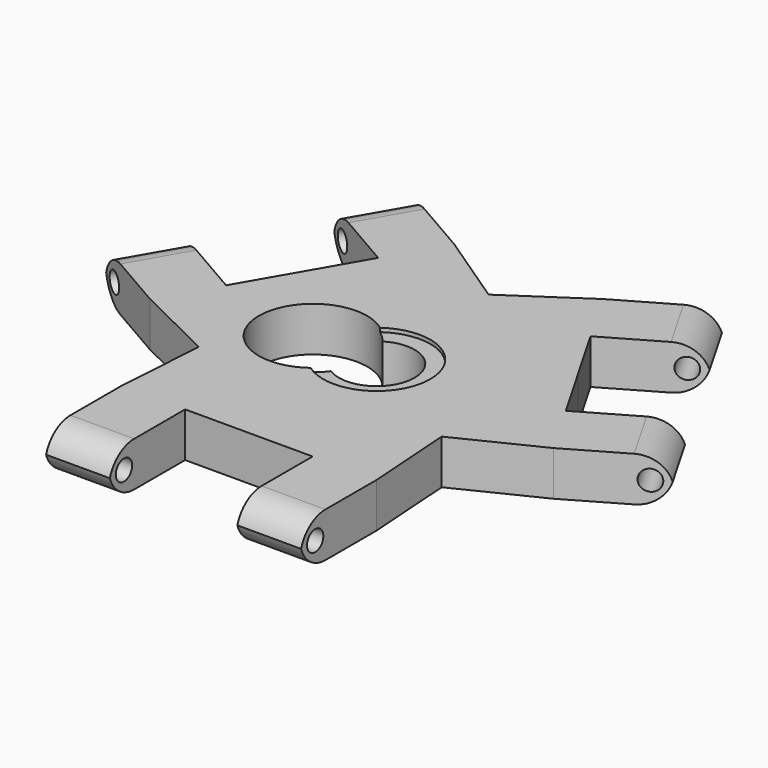
from build123d import *

# Parameters (mm, degrees)
F0_W         = 10
F0_H         = 15
F1_DEPTH     = 7
F3_DEPTH     = 60
F4_R         = 1.6
F5_DEPTH     = 60
F6_R         = 1.6
F7_DEPTH     = 60
F8_T1_DEPTH  = 35
F8_T3_DEPTH  = 35
F8_T5_DEPTH  = 35
F8_T7_DEPTH  = 35
F8_T9_DEPTH  = 35
F8_T11_DEPTH = 35
F11_DEPTH    = 25
F12_R        = 8.4
F13_DEPTH    = 0.6


# Not quite as in the source:
# - a fillet or chamfer that OpenCascade refuses, or shapes differently, is made with other operations: its cross-section is extruded or revolved along the edge and cut away or added
# - a feature names something its author has since deleted; it is built from what else it names


with BuildPart() as f1:
    # F0 (on Top) → F1 (new body)
    with BuildSketch(Plane.XY):
        Polygon((-19.0935776077, -11.020506829), (-0.0410187244, -0.020506829), (-21.6916538191, 12.479493171), (-26.6916538191, 3.8192391331), (-31.6916538191, -4.8410149047), align=None)
        Polygon((-0.0410187244, 21.979493171), (-0.0410187244, -0.020506829), (21.6096163702, 12.479493171), (16.6096163702, 21.1397472088), (11.6096163702, 29.8000012467), align=None)
        Polygon((19.0115401588, -11.020506829), (-0.0410187244, -0.020506829), (-0.0410187244, -25.020506829), (9.9589812756, -25.020506829), (19.9589812756, -25.020506829), align=None)
        Polygon((-0.0410187244, -25.020506829), (-0.0410187244, -0.020506829), (-19.0935776077, -11.020506829), (-20.0410187244, -25.020506829), (-10.0410187244, -25.020506829), align=None)
        Polygon((-21.6916538191, 12.479493171), (-0.0410187244, -0.020506829), (-0.0410187244, 21.979493171), (-11.6916538191, 29.8000012467), (-16.6916538191, 21.1397472088), align=None)
        Polygon((21.6096163702, 12.479493171), (-0.0410187244, -0.020506829), (19.0115401588, -11.020506829), (31.6096163702, -4.8410149047), (26.6096163702, 3.8192391331), align=None)
        Polygon((-29.6820348758, 28.6397472088), (-16.6916538191, 21.1397472088), (-11.6916538191, 29.8000012467), (-24.6820348758, 37.3000012467), align=None)
        Polygon((-31.6916538191, -4.8410149047), (-26.6916538191, 3.8192391331), (-39.6820348758, 11.3192391331), (-44.6820348758, 2.6589850953), align=None)
        Polygon((39.5999974269, 11.3192391331), (26.6096163702, 3.8192391331), (31.6096163702, -4.8410149047), (44.5999974269, 2.6589850953), align=None)
        Polygon((11.6096163702, 29.8000012467), (16.6096163702, 21.1397472088), (29.5999974269, 28.6397472088), (24.5999974269, 37.3000012467), align=None)
        with Locations((-15.0410187244, -32.520506829)):
            Rectangle(F0_W, F0_H)
        with Locations((14.9589812756, -32.520506829)):
            Rectangle(F0_W, F0_H)
    extrude(amount=F1_DEPTH)

    # F2 (on face) → F3 (cut)
    with BuildSketch(Plane.YZ.offset(19.9589812756)):
        with BuildLine():
            ThreePointArc((-35.420506829, 3.5), (-37.020506829, 5.1), (-38.620506829, 3.5))
            ThreePointArc((-38.620506829, 3.5), (-37.020506829, 1.9), (-35.420506829, 3.5))
        make_face()
    extrude(amount=-F3_DEPTH, mode=Mode.SUBTRACT)

    # F4 (on face) → F5 (cut)
    with BuildSketch(Plane(origin=(9.9986250363, -17.3181265688, 0), x_dir=(0.8660254038, 0.5, 0), z_dir=(0.5, -0.8660254038, 0))):
        with Locations((36.9542233281, 3.5)):
            Circle(F4_R)
    extrude(amount=-F5_DEPTH, mode=Mode.SUBTRACT)

    # F6 (on face) → F7 (cut)
    with BuildSketch(Plane(origin=(9.9808656014, 17.2873663252, 0), x_dir=(-0.8660254038, 0.5, 0), z_dir=(0.5, 0.8660254038, 0))):
        with Locations((37.0252698429, 3.5)):
            Circle(F6_R)
    extrude(amount=-F7_DEPTH, mode=Mode.SUBTRACT)

    # F8: fillet of radius 5 on 12 edges, made by hand

    # F8_s2 → F8_t1 (cut)
    with BuildSketch(Plane.YZ.offset(-32.5410187244)):
        with BuildLine():
            ThreePointArc((-35.020506829, 7), (-38.556040735, 5.5355339059), (-40.020506829, 2))
            Line((-40.020506829, 2), (-40.020506829, 7))
            Line((-40.020506829, 7), (-35.020506829, 7))
        make_face()
        with BuildLine():
            ThreePointArc((-35.020506829, 0), (-38.556040735, 1.4644660941), (-40.020506829, 5))
            Line((-40.020506829, 5), (-40.020506829, 0))
            Line((-40.020506829, 0), (-35.020506829, 0))
        make_face()
    extrude(amount=F8_T1_DEPTH, mode=Mode.SUBTRACT)

    # F8_s4 → F8_t3 (cut)
    with BuildSketch(Plane.YZ.offset(-2.5410187244)):
        with BuildLine():
            ThreePointArc((-35.020506829, 0), (-38.556040735, 1.4644660941), (-40.020506829, 5))
            Line((-40.020506829, 5), (-40.020506829, 0))
            Line((-40.020506829, 0), (-35.020506829, 0))
        make_face()
        with BuildLine():
            ThreePointArc((-35.020506829, 7), (-38.556040735, 5.5355339059), (-40.020506829, 2))
            Line((-40.020506829, 2), (-40.020506829, 7))
            Line((-40.020506829, 7), (-35.020506829, 7))
        make_face()
    extrude(amount=F8_T3_DEPTH, mode=Mode.SUBTRACT)

    # F8_s6 → F8_t5 (cut)
    with BuildSketch(Plane(origin=(16.2486250363, -28.1434441161, 0), x_dir=(0, 0, 1), z_dir=(-0.5, 0.8660254038, 0))):
        with BuildLine():
            ThreePointArc((7, 34.9542233281), (5.5355339059, 38.489757234), (2, 39.9542233281))
            Line((2, 39.9542233281), (7, 39.9542233281))
            Line((7, 39.9542233281), (7, 34.9542233281))
        make_face()
        with BuildLine():
            ThreePointArc((0, 34.9542233281), (1.4644660941, 38.489757234), (5, 39.9542233281))
            Line((5, 39.9542233281), (0, 39.9542233281))
            Line((0, 39.9542233281), (0, 34.9542233281))
        make_face()
    extrude(amount=F8_T5_DEPTH, mode=Mode.SUBTRACT)

    # F8_s8 → F8_t7 (cut)
    with BuildSketch(Plane(origin=(1.2486250363, -2.1626820025, 0), x_dir=(0, 0, 1), z_dir=(-0.5, 0.8660254038, 0))):
        with BuildLine():
            ThreePointArc((7, 34.9542233281), (5.5355339059, 38.489757234), (2, 39.9542233281))
            Line((2, 39.9542233281), (7, 39.9542233281))
            Line((7, 39.9542233281), (7, 34.9542233281))
        make_face()
        with BuildLine():
            ThreePointArc((0, 34.9542233281), (1.4644660941, 38.489757234), (5, 39.9542233281))
            Line((5, 39.9542233281), (0, 39.9542233281))
            Line((0, 39.9542233281), (0, 34.9542233281))
        make_face()
    extrude(amount=F8_T7_DEPTH, mode=Mode.SUBTRACT)

    # F8_s10 → F8_t9 (cut)
    with BuildSketch(Plane(origin=(16.2308656014, 28.1126838725, 0), x_dir=(0, 0, 1), z_dir=(-0.5, -0.8660254038, 0))):
        with BuildLine():
            ThreePointArc((7, 35.0252698429), (5.5355339059, 38.5608037488), (2, 40.0252698429))
            Line((2, 40.0252698429), (7, 40.0252698429))
            Line((7, 40.0252698429), (7, 35.0252698429))
        make_face()
        with BuildLine():
            ThreePointArc((0, 35.0252698429), (1.4644660941, 38.5608037488), (5, 40.0252698429))
            Line((5, 40.0252698429), (0, 40.0252698429))
            Line((0, 40.0252698429), (0, 35.0252698429))
        make_face()
    extrude(amount=F8_T9_DEPTH, mode=Mode.SUBTRACT)

    # F8_s12 → F8_t11 (cut)
    with BuildSketch(Plane(origin=(1.2308656014, 2.131921759, 0), x_dir=(0, 0, 1), z_dir=(-0.5, -0.8660254038, 0))):
        with BuildLine():
            ThreePointArc((7, 35.0252698429), (5.5355339059, 38.5608037488), (2, 40.0252698429))
            Line((2, 40.0252698429), (7, 40.0252698429))
            Line((7, 40.0252698429), (7, 35.0252698429))
        make_face()
        with BuildLine():
            ThreePointArc((0, 35.0252698429), (1.4644660941, 38.5608037488), (5, 40.0252698429))
            Line((5, 40.0252698429), (0, 40.0252698429))
            Line((0, 40.0252698429), (0, 35.0252698429))
        make_face()
    extrude(amount=F8_T11_DEPTH, mode=Mode.SUBTRACT)

    # F10 (on face) → F11 (cut)
    with BuildSketch(Plane.XY.offset(7)):
        with BuildLine():
            ThreePointArc((-3.157625, -5.0430054887), (-1.9250328948, -2.6542242275), (-1.5, 0))
            Line((-1.5, 0), (-5.95, 0))
            ThreePointArc((-5.95, 0), (-5.2053034854, -2.8822414238), (-3.157625, -5.0430054887))
        make_face()
        with BuildLine():
            Line((-5.95, 0), (-1.5, 0))
            ThreePointArc((-1.5, 0), (-1.9250328948, 2.6542242275), (-3.157625, 5.0430054887))
            ThreePointArc((-3.157625, 5.0430054887), (-5.2053034854, 2.8822414238), (-5.95, 0))
        make_face()
        with BuildLine():
            ThreePointArc((-3.157625, 5.0430054887), (-1.9250328948, 2.6542242275), (-1.5, 0))
            ThreePointArc((-1.5, 0), (-1.9250328948, -2.6542242275), (-3.157625, -5.0430054887))
            ThreePointArc((-3.157625, -5.0430054887), (2.8822414238, -5.2053034854), (5.95, 0))
            ThreePointArc((5.95, 0), (2.8822414238, 5.2053034854), (-3.157625, 5.0430054887))
        make_face()
        with BuildLine():
            ThreePointArc((-3.157625, -5.0430054887), (-5.2053034854, -2.8822414238), (-5.95, 0))
            ThreePointArc((-5.95, 0), (-5.2053034854, 2.8822414238), (-3.157625, 5.0430054887))
            ThreePointArc((-3.157625, 5.0430054887), (-18.5, 0), (-3.157625, -5.0430054887))
        make_face()
    extrude(amount=-F11_DEPTH, mode=Mode.SUBTRACT)

    # F12 (on face) → F13 (cut)
    with BuildSketch(Plane.XY.offset(7)):
        Circle(F12_R)
    extrude(amount=-F13_DEPTH, mode=Mode.SUBTRACT)


solid = f1.part
